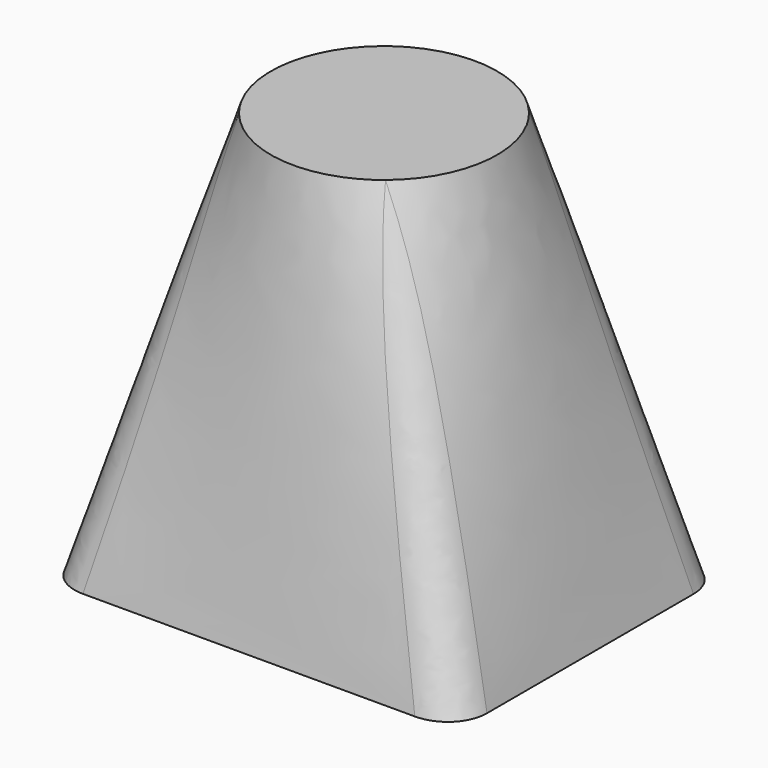
from build123d import *

# Parameters (mm, degrees)
F0_W = 50.4621304572
F0_H = 41.2473119795
F4_R = 5


# Not quite as in the source:
# - the arcs of a loft's sections are written as splines that run evenly, so that the points pair up as in the source's solid


with BuildPart() as f3:
    # F0 (on Top) → F3 section 0
    with BuildSketch(Plane.XY):
        Rectangle(F0_W, F0_H)
    # F2 (on offset) → F3 section 1
    with BuildSketch(Plane.XY.offset(50)):
        with BuildLine():
            add(Edge.make_bspline(
                [(10.7235170513, 8.7653107256), (9.5761405604, 10.1690158252), (8.1501110676, 11.3440310504), (4.9556863845, 13.0595759251), (3.1885480639, 13.5994305811), (-0.4192261201, 13.9619339759), (-2.2584424784, 13.784440085), (-5.7303152482, 12.738714144), (-7.3616056261, 11.8708935423), (-8.7653107256, 10.7235170513)],
                knots=[0, 0, 0, 0, 0.25, 0.25, 0.5, 0.5, 0.75, 0.75, 1, 1, 1, 1], degree=3))
            add(Edge.make_bspline(
                [(-8.7653107256, 10.7235170513), (-10.1690158252, 9.5761405604), (-11.3440310504, 8.1501110676), (-13.0595759251, 4.9556863845), (-13.5994305811, 3.1885480639), (-13.9619339759, -0.4192261201), (-13.784440085, -2.2584424784), (-12.738714144, -5.7303152482), (-11.8708935423, -7.3616056261), (-10.7235170513, -8.7653107256)],
                knots=[0, 0, 0, 0, 0.25, 0.25, 0.5, 0.5, 0.75, 0.75, 1, 1, 1, 1], degree=3))
            add(Edge.make_bspline(
                [(-10.7235170513, -8.7653107256), (-9.5761405604, -10.1690158252), (-8.1501110676, -11.3440310504), (-4.9556863845, -13.0595759251), (-3.1885480639, -13.5994305811), (0.4192261201, -13.9619339759), (2.2584424784, -13.784440085), (5.7303152482, -12.738714144), (7.3616056261, -11.8708935423), (8.7653107256, -10.7235170513)],
                knots=[0, 0, 0, 0, 0.25, 0.25, 0.5, 0.5, 0.75, 0.75, 1, 1, 1, 1], degree=3))
            add(Edge.make_bspline(
                [(8.7653107256, -10.7235170513), (10.1690158252, -9.5761405604), (11.3440310504, -8.1501110676), (13.0595759251, -4.9556863845), (13.5994305811, -3.1885480639), (13.9619339759, 0.4192261201), (13.784440085, 2.2584424784), (12.738714144, 5.7303152482), (11.8708935423, 7.3616056261), (10.7235170513, 8.7653107256)],
                knots=[0, 0, 0, 0, 0.25, 0.25, 0.5, 0.5, 0.75, 0.75, 1, 1, 1, 1], degree=3))
        make_face()
    loft(ruled=True)

    # F4
    f4_edges = [f3.edges().sort_by_distance(p)[0] for p in [
        (17.977291, 14.694483, 25),
        (16.998188, -15.673587, 25),
        (-16.998188, 15.673587, 25),
        (-17.977291, -14.694483, 25),
    ]]
    fillet(f4_edges, radius=F4_R)


solid = f3.part
